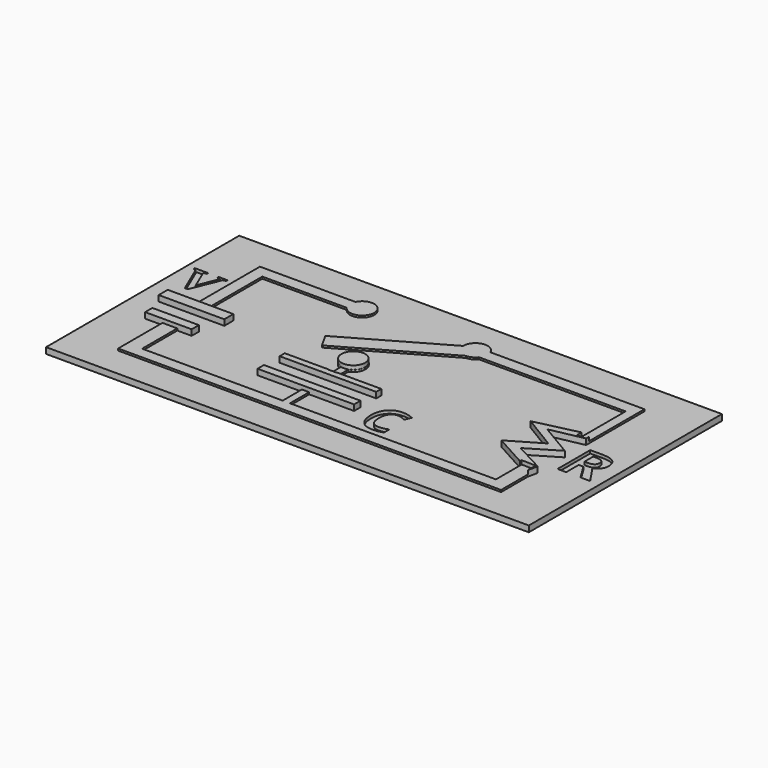
from build123d import *

# Parameters (mm, degrees)
F0_W            = 127
F0_H            = 63.5
F1_DEPTH        = 1.5875
F3_DEPTH        = 0.508
F5_DEPTH        = 1.524
F7_DEPTH        = 1.524
F9_DEPTH        = 1.524
F10_TEXT_SIZE   = 13.4132621396
F10_TEXT_SIZE_2 = 15.0686647329
F10_TEXT_SIZE_3 = 12.2738122526
F11_DEPTH       = 0.79375
F12_R           = 3.1292851238
F13_DEPTH       = 1.016


# Not quite as in the source:
# - Text() gives the source's letters only with a copy of the font that has no kerning and outlines rounded to 1/6400 em; it was checked with that copy


with BuildPart() as f1:
    # F0 (on Top) → F1 (new body)
    with BuildSketch(Plane.XY):
        with Locations((63.5, 31.75)):
            Rectangle(F0_W, F0_H)
    extrude(amount=F1_DEPTH)

    # F2 (on face) → F3 (join)
    with BuildSketch(Plane.XY.offset(1.5875)):
        with BuildLine():
            Line((15.6837590039, 51.4970384538), (37.9034765019, 51.4970384538))
            ThreePointArc((37.9034765019, 51.4970384538), (43.701255331, 53.5076912736), (37.6708468588, 54.6439737082))
            Line((37.6708468588, 54.6439737082), (12.5394938514, 54.6439737082))
            Line((12.5394938514, 54.6439737082), (12.5394938514, 33.2438908517))
            Line((12.5394938514, 33.2438908517), (15.6837590039, 33.2438908517))
            Line((15.6837590039, 33.2438908517), (15.6837590039, 51.4970384538))
        make_face()
        with BuildLine():
            Line((44.3884748903, 35.2514416882), (70.3707262874, 50.0986256719))
            ThreePointArc((70.3707262874, 50.0986256719), (71.7473772471, 50.4126018804), (72.8517537823, 51.2924322009))
            Line((72.8517537823, 51.2924322009), (111.4279255271, 51.2924322009))
            Line((111.4279255271, 51.2924322009), (111.4279255271, 35.2854765952))
            Line((111.4279255271, 35.2854765952), (113.6307865381, 35.2854765952))
            Line((113.6307865381, 35.2854765952), (113.8216480613, 35.2854765952))
            Line((113.8216480613, 35.2854765952), (113.8481348753, 36.1864678562))
            Line((113.8481348753, 36.1864678562), (113.8481348753, 54.4674322009))
            Line((113.8481348753, 54.4674322009), (73.3127410683, 54.4674322009))
            ThreePointArc((73.3127410683, 54.4674322009), (69.7247921245, 56.3822256875), (67.1966613405, 53.1965756033))
            Line((67.1966613405, 53.1965756033), (57.5713776052, 47.7047674358))
            Line((57.5713776052, 47.7047674358), (42.2656994117, 38.9719497003))
            Line((42.2656994117, 38.9719497003), (44.3884748903, 35.2514416882))
        make_face()
        with BuildLine():
            Line((55.3403832018, 26.1289812624), (55.3403832018, 30.2673894981))
            ThreePointArc((55.3403832018, 30.2673894981), (54.0820823428, 36.4151885913), (53.422562778, 30.1746927228))
            Line((53.422562778, 30.1746927228), (53.422562778, 26.1289812624))
            Line((53.422562778, 26.1289812624), (55.3403832018, 26.1289812624))
        make_face()
        Polygon((16.4452474564, 22.5945748389), (12.5394938514, 22.5945748389), (12.5394938514, 8.0218240619), (113.2876425982, 8.0218240619), (113.2876425982, 19.3717554212), (109.5263585448, 19.4896757603), (109.5263585448, 11.0277580097), (55.3403832018, 11.0277580097), (55.3403832018, 17.3531314358), (53.422562778, 17.3531314358), (53.422562778, 11.0277580097), (16.4452474564, 11.0277580097), align=None)
    extrude(amount=F3_DEPTH)

    # F4 (on face) → F5 (join)
    with BuildSketch(Plane.XY.offset(1.5875)):
        Polygon((105.0436720252, 33.4897376597), (113.8481348753, 35.2854765952), (113.8481348753, 36.1864678562), (113.8216480613, 35.2854765952), (111.4279255271, 35.2854765952), (111.4279255271, 36.8072942313), (100.1392528415, 34.1735742986), (109.1646552086, 28.6978967488), (100.7789373398, 23.7623024732), (109.5263585448, 18.9372065652), (109.5263585448, 19.4896757603), (113.2876425982, 19.3717554212), (113.2876425982, 16.8624743819), (113.8481348753, 19.3717554212), (105.9792414308, 23.5563572496), (113.8481348753, 28.2666310668), align=None)
    extrude(amount=F5_DEPTH)

    # F6 (on face) → F7 (join)
    with BuildSketch(Plane.XY.offset(1.5875)):
        Polygon((12.5394938514, 33.2438908517), (5.4079336114, 33.2438908517), (5.4079336114, 30.2680805326), (22.6676166058, 30.2680805326), (22.6676166058, 33.2438908517), (15.6837590039, 33.2438908517), align=None)
        Polygon((20.2208422124, 24.9752197415), (7.9869665205, 24.9752197415), (7.9869665205, 22.5945748389), (12.5394938514, 22.5945748389), (16.4452474564, 22.5945748389), (20.2208422124, 22.5945748389), align=None)
    extrude(amount=F7_DEPTH)

    # F8 (on face) → F9 (join)
    with BuildSketch(Plane.XY.offset(1.5875)):
        Polygon((53.422562778, 26.2253240671), (41.8131047737, 26.2253240671), (41.8131047737, 24.5413463212), (67.2131047737, 24.5413463212), (67.2131047737, 26.2253240671), (55.3403832018, 26.2253240671), (55.3403832018, 26.1289812624), (53.422562778, 26.1289812624), align=None)
        Polygon((67.1429432273, 19.4581050173), (41.7429432273, 19.4581050173), (41.7429432273, 17.3531314358), (53.422562778, 17.3531314358), (55.3403832018, 17.3531314358), (67.1429432273, 17.3531314358), align=None)
    extrude(amount=F9_DEPTH)

    # F10 (on face) → F11 (cut)
    with BuildSketch(Plane.XY.offset(1.5875)):
        with Locations((70.2249726593, 13.3567433804)):
            Text('C', F10_TEXT_SIZE, font='Open Sans', font_style=FontStyle.BOLD, text_align=(TextAlign.LEFT, TextAlign.BOTTOM))
        with Locations((114.5433187485, 23.306068033)):
            Text('R', F10_TEXT_SIZE_2, font='Open Sans', font_style=FontStyle.BOLD, text_align=(TextAlign.LEFT, TextAlign.BOTTOM))
        with Locations((1.7807033146, 38.4911671281)):
            Text('V', F10_TEXT_SIZE_3, font='Tinos', font_style=FontStyle.BOLD, text_align=(TextAlign.LEFT, TextAlign.BOTTOM))
    extrude(amount=-F11_DEPTH, mode=Mode.SUBTRACT)

    # F12 (on face) → F13 (join)
    with BuildSketch(Plane.XY.offset(2.0955)):
        with Locations((54.2353652418, 33.2438908517)):
            Circle(F12_R)
    extrude(amount=F13_DEPTH)


solid = f1.part
